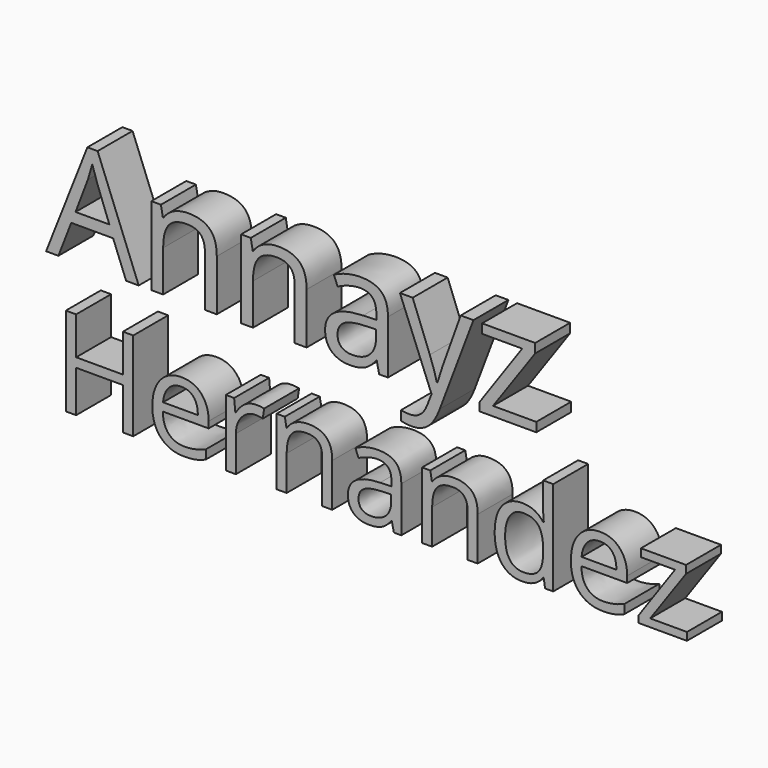
from build123d import *

# Parameters (mm, degrees)
F0_TEXT_SIZE   = 85.0750081655
F0_TEXT_SIZE_2 = 72.2730273588
F1_DEPTH       = 25.4


# Not quite as in the source:
# - Text() gives the source's letters only with a copy of the font that has no kerning and outlines rounded to 1/6400 em; it was checked with that copy


with BuildPart() as f1:
    # F0 (on Front) → F1 (new body)
    with BuildSketch(Plane.XZ):
        with Locations((-130.7375580072, 0)):
            Text('Annayz', F0_TEXT_SIZE, font='Open Sans', text_align=(TextAlign.LEFT, TextAlign.BOTTOM))
        with Locations((-126.3591051102, -78.2052651048)):
            Text('Hernandez', F0_TEXT_SIZE_2, font='Open Sans', text_align=(TextAlign.LEFT, TextAlign.BOTTOM))
    extrude(amount=F1_DEPTH)


solid = f1.part
